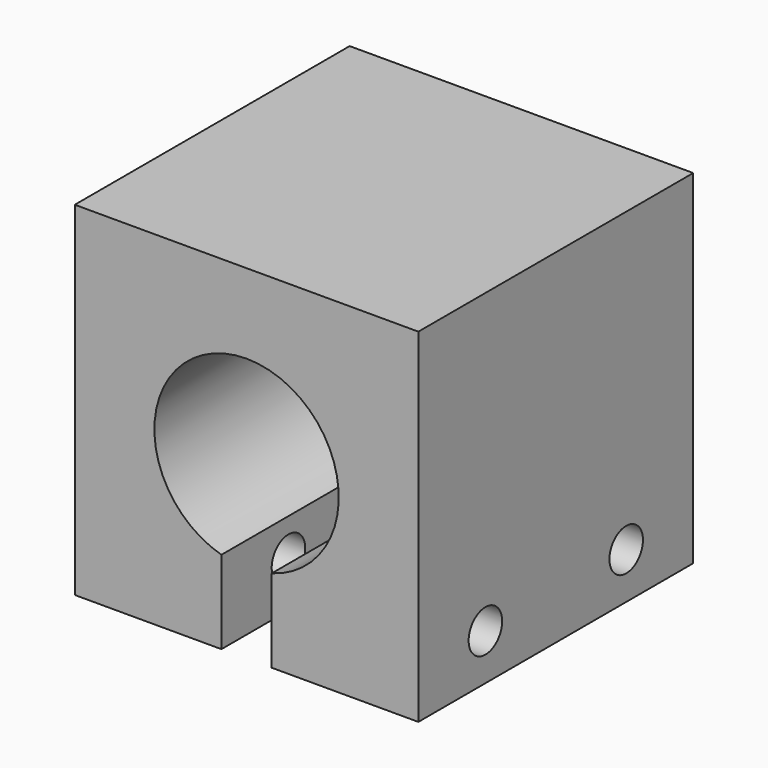
from build123d import *

# Parameters (mm, degrees)
F0_W     = 41
F0_H     = 41
F0_R     = 11
F1_DEPTH = 41
F2_W     = 6
F2_H     = 11.5
F3_DEPTH = 41.001
F4_R     = 2.5
F5_DEPTH = 41.001


# Not quite as in the source:
# - a feature names something its author has since deleted; it is built from what else it names


with BuildPart() as f1:
    # F0 (on Front) → F1 (new body)
    with BuildSketch(Plane.XZ):
        Rectangle(F0_W, F0_H)
        Circle(F0_R, mode=Mode.SUBTRACT)
    extrude(amount=F1_DEPTH)

    # F2 (on Front) → F3 (cut, through all)
    with BuildSketch(Plane.XZ):
        with Locations((0, -14.9551387876)):
            Rectangle(F2_W, F2_H)
    extrude(amount=F3_DEPTH, mode=Mode.SUBTRACT)

    # F4 (on face) → F5 (cut, through all)
    with BuildSketch(Plane.YZ.offset(20.5)):
        with Locations((-31, -15)):
            Circle(F4_R)
        with Locations((-10, -15)):
            Circle(F4_R)
    extrude(amount=-F5_DEPTH, mode=Mode.SUBTRACT)


solid = f1.part
